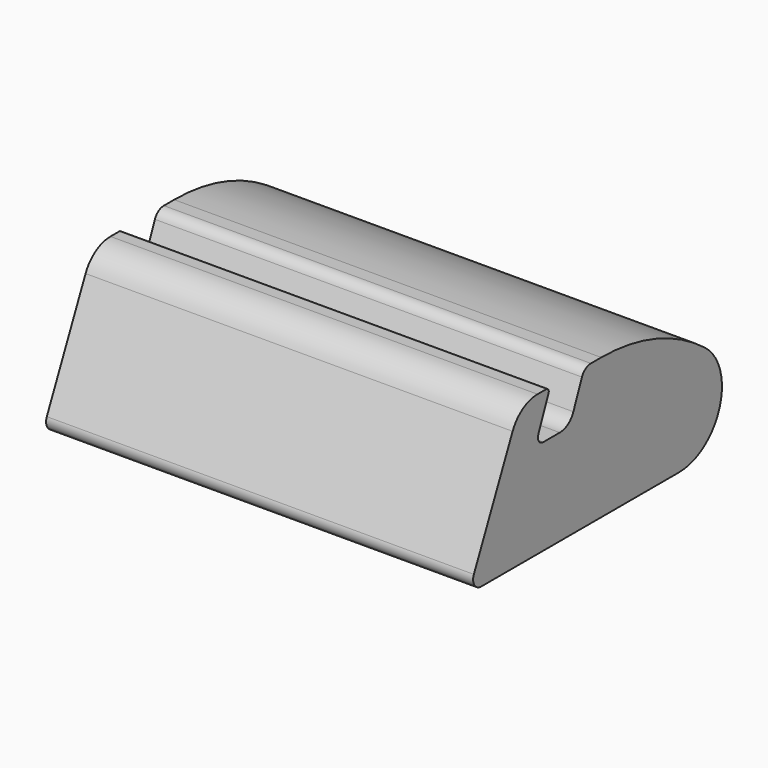
from build123d import *

# Parameters (mm, degrees)
F1_DEPTH    = 63.5
F2_R        = 1.7934980513
F3_R        = 0.4788394015
F4_R        = 2.7306448225
F5_R        = 0.9937962324
F6_R        = 5.08
F7_R        = 1.519546052
F8_T1_DEPTH = 212.3191575165
F9_R        = 7.9959076321


# Not quite as in the source:
# - a fillet or chamfer that OpenCascade refuses, or shapes differently, is made with other operations: its cross-section is extruded or revolved along the edge and cut away or added


with BuildPart() as f1:
    # F0 (on Right) → F1 (new body)
    with BuildSketch(Plane.YZ):
        Polygon((-16.9031135738, 20.9204703569), (-26.4463126659, 0), (27.971111238, 0), (27.971111238, 20.9204703569), (-4.9152970314, 20.9204703569), (-7.6606271703, 14.2183713615), (-14.0469465405, 14.2183713615), (-11.3016164016, 20.9204703569), align=None)
    extrude(amount=F1_DEPTH)

    # F2
    f2_edges = [f1.edges().sort_by_distance(p)[0] for p in [
        (31.75, -4.915297, 20.92047),
    ]]
    fillet(f2_edges, radius=F2_R)

    # F3
    f3_edges = [f1.edges().sort_by_distance(p)[0] for p in [
        (31.75, -11.301616, 20.92047),
    ]]
    fillet(f3_edges, radius=F3_R)

    # F4
    f4_edges = [f1.edges().sort_by_distance(p)[0] for p in [
        (31.75, -7.660627, 14.218371),
    ]]
    fillet(f4_edges, radius=F4_R)

    # F5
    f5_edges = [f1.edges().sort_by_distance(p)[0] for p in [
        (31.75, -14.046947, 14.218371),
    ]]
    fillet(f5_edges, radius=F5_R)

    # F6
    f6_edges = [f1.edges().sort_by_distance(p)[0] for p in [
        (31.75, -16.903114, 20.92047),
    ]]
    fillet(f6_edges, radius=F6_R)

    # F7
    f7_edges = [f1.edges().sort_by_distance(p)[0] for p in [
        (31.75, -26.446313, 0),
    ]]
    fillet(f7_edges, radius=F7_R)

    # F8: fillet of radius 31.6329347077 on 1 edges, made by hand

    # F8_s2 → F8_t1 (cut)
    with BuildSketch(Plane.YZ.offset(-74.4095787583)):
        with BuildLine():
            ThreePointArc((27.971111238, 0), (16.3976050872, 15.1671535327), (-1.7927202653, 20.9204703569))
            Line((-1.7927202653, 20.9204703569), (27.971111238, 20.9204703569))
            Line((27.971111238, 20.9204703569), (27.971111238, 0))
        make_face()
    extrude(amount=F8_T1_DEPTH, mode=Mode.SUBTRACT)

    # F9
    f9_edges = [f1.edges().sort_by_distance(p)[0] for p in [
        (31.75, 27.971111, 0),
    ]]
    fillet(f9_edges, radius=F9_R)


solid = f1.part
